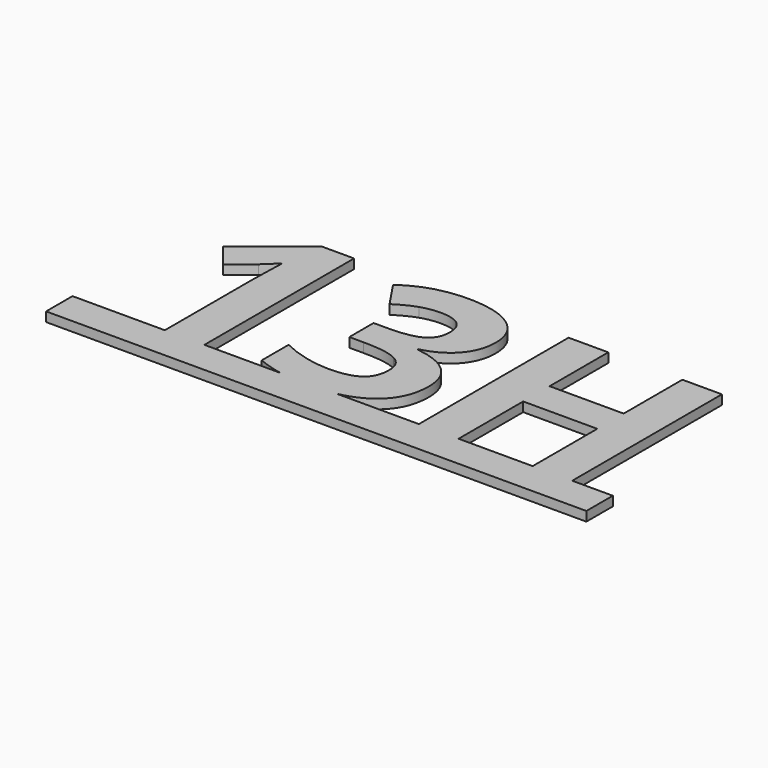
from build123d import *

# Parameters (mm, degrees)
F1_DEPTH = 50.8


# Not quite as in the source:
# - a feature names something its author has since deleted; it is built from what else it names


with BuildPart() as f1:
    # F0 (on Top) → F1 (new body)
    with BuildSketch(Plane.XY):
        with BuildLine():
            Line((-362.7747852802, 0), (-362.7747852802, -177.8))
            Line((-362.7747852802, -177.8), (2545.8779924975, -177.8))
            Line((2545.8779924975, -177.8), (2545.8779924975, 0))
            Line((2545.8779924975, 0), (2327.3762563864, 0))
            Line((2327.3762563864, 0), (2114.3866730531, 0))
            Line((2114.3866730531, 0), (1715.5272980531, 0))
            Line((1715.5272980531, 0), (1501.8762563864, 0))
            Line((1501.8762563864, 0), (1060.7698674064, 0))
            add(Edge.make_bspline(
                [(1060.7698674064, 0), (995.2549319361, -13.890625), (914.2807702753, -13.890625)],
                knots=[0.5859606644, 0.5859606644, 0.5859606644, 1, 1, 1], degree=2))
            add(Edge.make_bspline(
                [(914.2807702753, -13.890625), (831.4339258388, -13.890625), (758.0911932443, 0)],
                knots=[0, 0, 0, 0.5050353738, 0.5050353738, 0.5050353738], degree=2))
            Line((758.0911932443, 0), (347.1904924976, 0))
            Line((347.1904924976, 0), (134.2009091642, 0))
            Line((134.2009091642, 0), (-362.7747852802, 0))
        make_face()
        with BuildLine():
            Line((1060.7698674064, 0), (758.0911932443, 0))
            add(Edge.make_bspline(
                [(914.2807702753, -13.890625), (831.4339258388, -13.890625), (758.0911932443, 0)],
                knots=[0, 0, 0, 0.5050353738, 0.5050353738, 0.5050353738], degree=2))
            add(Edge.make_bspline(
                [(1060.7698674064, 0), (995.2549319361, -13.890625), (914.2807702753, -13.890625)],
                knots=[0.5859606644, 0.5859606644, 0.5859606644, 1, 1, 1], degree=2))
        make_face()
        with BuildLine():
            add(Edge.make_bspline(
                [(758.0911932443, 0), (686.2109644272, 13.6136365267), (623.4595897198, 40.5694444444)],
                knots=[0.5050353738, 0.5050353738, 0.5050353738, 1, 1, 1], degree=2))
            Line((758.0911932443, 0), (1060.7698674064, 0))
            add(Edge.make_bspline(
                [(1215.244311942, 67.1380208333), (1153.4885340032, 19.6584216858), (1060.7698674064, 0)],
                knots=[0, 0, 0, 0.5859606644, 0.5859606644, 0.5859606644], degree=2))
            add(Edge.make_bspline(
                [(1320.6366730531, 293.4670138889), (1320.6366730531, 148.1666666667), (1215.244311942, 67.1380208333)],
                knots=[0, 0, 0, 1, 1, 1], degree=2))
            add(Edge.make_bspline(
                [(1258.0186174976, 452.3272569444), (1320.6366730531, 393.3472222222), (1320.6366730531, 293.4670138889)],
                knots=[0, 0, 0, 1, 1, 1], degree=2))
            add(Edge.make_bspline(
                [(1073.2512563864, 526.5208333333), (1195.400561942, 511.3072916667), (1258.0186174976, 452.3272569444)],
                knots=[0, 0, 0, 1, 1, 1], degree=2))
            Line((1073.2512563864, 526.5208333333), (1073.2512563864, 530.4895833333))
            add(Edge.make_bspline(
                [(1233.8753883309, 621.5503472222), (1176.6592424976, 555.4045138889), (1073.2512563864, 530.4895833333)],
                knots=[0, 0, 0, 1, 1, 1], degree=2))
            add(Edge.make_bspline(
                [(1291.0915341642, 782.0642361111), (1291.0915341642, 687.6961805556), (1233.8753883309, 621.5503472222)],
                knots=[0, 0, 0, 1, 1, 1], degree=2))
            add(Edge.make_bspline(
                [(1200.4717424976, 958.3428819444), (1291.0915341642, 894.953125), (1291.0915341642, 782.0642361111)],
                knots=[0, 0, 0, 1, 1, 1], degree=2))
            add(Edge.make_bspline(
                [(953.5272980531, 1021.7326388889), (1109.8519508309, 1021.7326388889), (1200.4717424976, 958.3428819444)],
                knots=[0, 0, 0, 1, 1, 1], degree=2))
            add(Edge.make_bspline(
                [(624.7825063864, 922.5138888889), (762.5863258309, 1021.7326388889), (953.5272980531, 1021.7326388889)],
                knots=[0, 0, 0, 1, 1, 1], degree=2))
            Line((624.7825063864, 922.5138888889), (723.3397980531, 775.890625))
            add(Edge.make_bspline(
                [(837.3311174976, 832.9965277778), (785.9578536087, 816.4600694444), (723.3397980531, 775.890625)],
                knots=[0, 0, 0, 1, 1, 1], degree=2))
            add(Edge.make_bspline(
                [(938.3137563864, 849.5329861111), (888.7043813864, 849.5329861111), (837.3311174976, 832.9965277778)],
                knots=[0, 0, 0, 1, 1, 1], degree=2))
            add(Edge.make_bspline(
                [(1081.6297286087, 735.1006944444), (1081.6297286087, 849.5329861111), (938.3137563864, 849.5329861111)],
                knots=[0, 0, 0, 1, 1, 1], degree=2))
            add(Edge.make_bspline(
                [(1027.5003883309, 630.1493055556), (1081.6297286087, 660.796875), (1081.6297286087, 735.1006944444)],
                knots=[0, 0, 0, 1, 1, 1], degree=2))
            add(Edge.make_bspline(
                [(856.2929230531, 599.5017361111), (973.3710480531, 599.5017361111), (1027.5003883309, 630.1493055556)],
                knots=[0, 0, 0, 1, 1, 1], degree=2))
            Line((856.2929230531, 599.5017361111), (778.4613258309, 599.5017361111))
            Line((778.4613258309, 599.5017361111), (778.4613258309, 436.1215277778))
            Line((778.4613258309, 436.1215277778), (854.9700063864, 436.1215277778))
            add(Edge.make_bspline(
                [(1039.627124442, 406.4661458333), (981.7495202753, 436.1215277778), (854.9700063864, 436.1215277778)],
                knots=[0, 0, 0, 1, 1, 1], degree=2))
            add(Edge.make_bspline(
                [(1097.5047286087, 306.0347222222), (1097.5047286087, 376.8107638889), (1039.627124442, 406.4661458333)],
                knots=[0, 0, 0, 1, 1, 1], degree=2))
            add(Edge.make_bspline(
                [(1047.2338952753, 190.8307291667), (1097.5047286087, 226.6597222222), (1097.5047286087, 306.0347222222)],
                knots=[0, 0, 0, 1, 1, 1], degree=2))
            add(Edge.make_bspline(
                [(891.3502147198, 155.0017361111), (996.963061942, 155.0017361111), (1047.2338952753, 190.8307291667)],
                knots=[0, 0, 0, 1, 1, 1], degree=2))
            add(Edge.make_bspline(
                [(752.2234786087, 173.6328125), (822.5585480531, 155.0017361111), (891.3502147198, 155.0017361111)],
                knots=[0, 0, 0, 1, 1, 1], degree=2))
            add(Edge.make_bspline(
                [(623.4595897198, 221.8090277778), (681.8884091642, 192.2638888889), (752.2234786087, 173.6328125)],
                knots=[0, 0, 0, 1, 1, 1], degree=2))
            Line((623.4595897198, 221.8090277778), (623.4595897198, 40.5694444444))
        make_face()
        Polygon((2114.3866730531, 0), (2327.3762563864, 0), (2327.3762563864, 1007.4010416667), (2114.3866730531, 1007.4010416667), (2114.3866730531, 612.5104166667), (1715.5272980531, 612.5104166667), (1715.5272980531, 1007.4010416667), (1501.8762563864, 1007.4010416667), (1501.8762563864, 0), (1715.5272980531, 0), (1715.5272980531, 434.7986111111), (2114.3866730531, 434.7986111111), align=None)
        with BuildLine():
            Line((134.2009091642, 582.9652777778), (134.2009091642, 0))
            Line((134.2009091642, 0), (347.1904924976, 0))
            Line((347.1904924976, 0), (347.1904924976, 1007.4010416667))
            Line((347.1904924976, 1007.4010416667), (172.1245202753, 1007.4010416667))
            Line((172.1245202753, 1007.4010416667), (-152.4310352802, 748.9913194444))
            Line((-152.4310352802, 748.9913194444), (-49.6845075024, 620.8888888889))
            Line((-49.6845075024, 620.8888888889), (66.0707008309, 713.9340277778))
            add(Edge.make_bspline(
                [(139.713061942, 783.3871527778), (86.7963952753, 730.4704861111), (66.0707008309, 713.9340277778)],
                knots=[0, 0, 0, 1, 1, 1], degree=2))
            Line((139.713061942, 783.3871527778), (136.4057702753, 678.65625))
            Line((136.4057702753, 678.65625), (134.2009091642, 582.9652777778))
        make_face()
    extrude(amount=F1_DEPTH)


solid = f1.part
